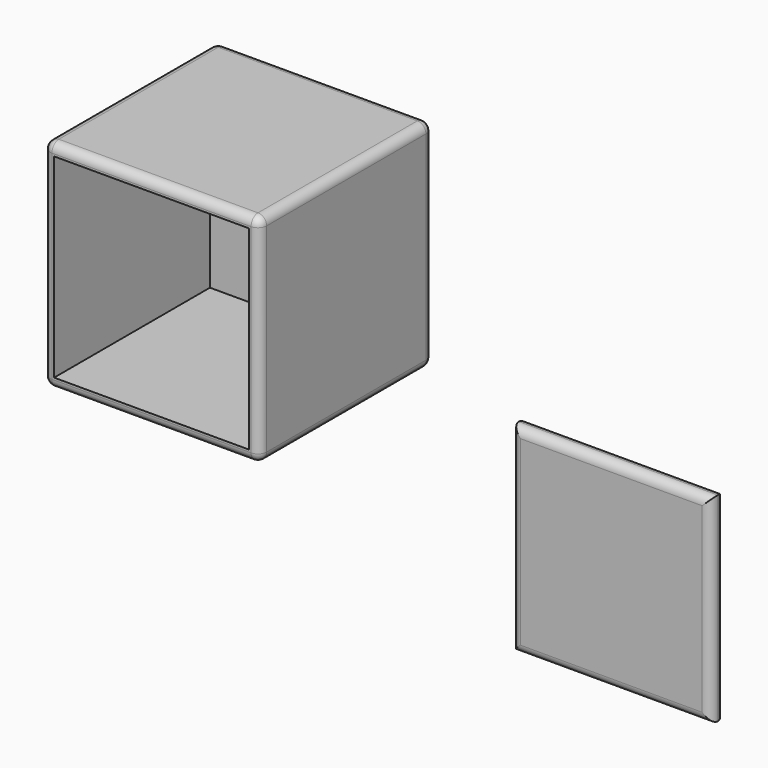
from build123d import *

# Parameters (mm, degrees)
F0_W     = 127
F0_H     = 127
F1_DEPTH = 127
F0_W_2   = 116.84
F0_H_2   = 116.84
F2_DEPTH = 10.16
F3_R     = 5.08
F4_W     = 114.3
F4_H     = 114.3
F5_DEPTH = 114.3
F6_R     = 5.08
F7_R     = 5.07999


# Not quite as in the source:
# - a fillet or chamfer is up to 0.001 mm smaller than in the source, because OpenCascade refuses the exact size


with BuildPart() as f1:
    # F0 (on Front) → F1 (new body)
    with BuildSketch(Plane.XZ):
        with Locations((-66.5750936817, 53.7270531058)):
            Rectangle(F0_W, F0_H)
    extrude(amount=F1_DEPTH)

    # F4 (on face) → F5 (cut)
    with BuildSketch(Plane.XZ.offset(127)):
        with Locations((-66.5750936817, 53.7270531058)):
            Rectangle(F4_W, F4_H)
    extrude(amount=-F5_DEPTH, mode=Mode.SUBTRACT)

    # F6
    f6_edges = [f1.edges().sort_by_distance(p)[0] for p in [
        (-130.075094, -63.5, -9.772947),
        (-3.075094, -63.5, -9.772947),
        (-66.575094, 0, -9.772947),
        (-66.575094, -127, -9.772947),
        (-130.075094, -63.5, 117.227053),
        (-130.075094, 0, 53.727053),
        (-130.075094, -127, 53.727053),
        (-3.075094, -63.5, 117.227053),
        (-3.075094, 0, 53.727053),
        (-3.075094, -127, 53.727053),
        (-66.575094, 0, 117.227053),
        (-66.575094, -127, 117.227053),
    ]]
    fillet(f6_edges, radius=F6_R)


with BuildPart() as f2:
    # F0 (on Front) → F2 (new body)
    with BuildSketch(Plane.XZ):
        with Locations((109.7554949653, -77.1886917222)):
            Rectangle(F0_W_2, F0_H_2)
    extrude(amount=F2_DEPTH)

    # F3
    f3_edges = [f2.edges().sort_by_distance(p)[0] for p in [
        (109.755495, -10.16, -18.768692),
        (51.335495, -10.16, -77.188692),
        (109.755495, -10.16, -135.608692),
        (168.175495, -10.16, -77.188692),
    ]]
    fillet(f3_edges, radius=F3_R)

    # F7 (radius 5.08 in the source; OpenCascade refuses exactly that, so slightly less here)
    f7_edges = [f2.edges().sort_by_distance(p)[0] for p in [
        (109.755495, 0, -18.768692),
        (51.335495, 0, -77.188692),
        (109.755495, 0, -135.608692),
        (168.175495, 0, -77.188692),
    ]]
    fillet(f7_edges, radius=F7_R)


solid = Compound([f1.part, f2.part])
